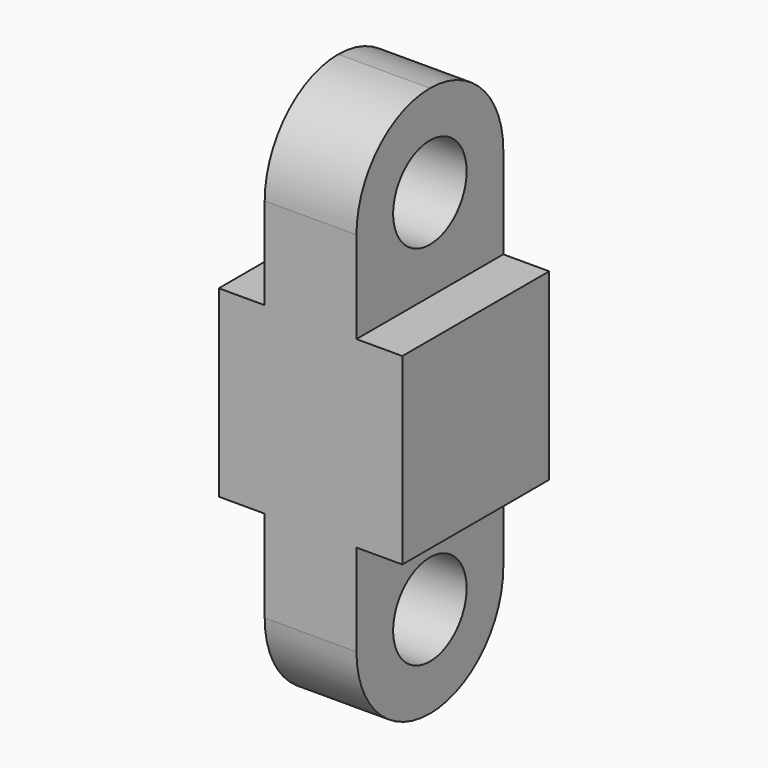
from build123d import *

# Parameters (mm, degrees)
F0_W      = 40
F0_H      = 120
F1_DEPTH  = 40
F2_W      = 10
F2_H      = 40
F3_DEPTH  = 40
F4_W      = 10
F4_H      = 40
F5_DEPTH  = 40
F6_W      = 10
F6_H      = 40
F7_DEPTH  = 40
F8_R      = 10
F9_DEPTH  = 25
F10_R     = 10
F11_DEPTH = 25
F12_R     = 19.99999


# Not quite as in the source:
# - a fillet or chamfer is up to 0.001 mm smaller than in the source, because OpenCascade refuses the exact size


with BuildPart() as f1:
    # F0 (on Front) → F1 (new body)
    with BuildSketch(Plane.XZ):
        Rectangle(F0_W, F0_H)
    extrude(amount=F1_DEPTH)

    # F2 (on face) → F3 (cut)
    with BuildSketch(Plane.XZ.offset(40)):
        with Locations((-15, 40)):
            Rectangle(F2_W, F2_H)
    extrude(amount=-F3_DEPTH, mode=Mode.SUBTRACT)

    # F4 (on face) → F5 (cut)
    with BuildSketch(Plane.XZ.offset(40)):
        with Locations((15, 40)):
            Rectangle(F4_W, F4_H)
    extrude(amount=-F5_DEPTH, mode=Mode.SUBTRACT)

    # F6 (on face) → F7 (cut)
    with BuildSketch(Plane.XZ.offset(40)):
        with Locations((-15, -40)):
            Rectangle(F6_W, F6_H)
        with Locations((15, -40)):
            Rectangle(F6_W, F6_H)
    extrude(amount=-F7_DEPTH, mode=Mode.SUBTRACT)

    # F8 (on face) → F9 (cut)
    with BuildSketch(Plane.YZ.offset(10)):
        with Locations((-20, 40)):
            Circle(F8_R)
    extrude(amount=-F9_DEPTH, mode=Mode.SUBTRACT)

    # F10 (on face) → F11 (cut)
    with BuildSketch(Plane.YZ.offset(10)):
        with Locations((-20, -40)):
            Circle(F10_R)
    extrude(amount=-F11_DEPTH, mode=Mode.SUBTRACT)

    # F12 (radius 20 in the source; OpenCascade refuses exactly that, so slightly less here)
    f12_edges = [f1.edges().sort_by_distance(p)[0] for p in [
        (0, -40, 60),
        (0, 0, 60),
        (0, -40, -60),
        (0, 0, -60),
    ]]
    fillet(f12_edges, radius=F12_R)


solid = f1.part
